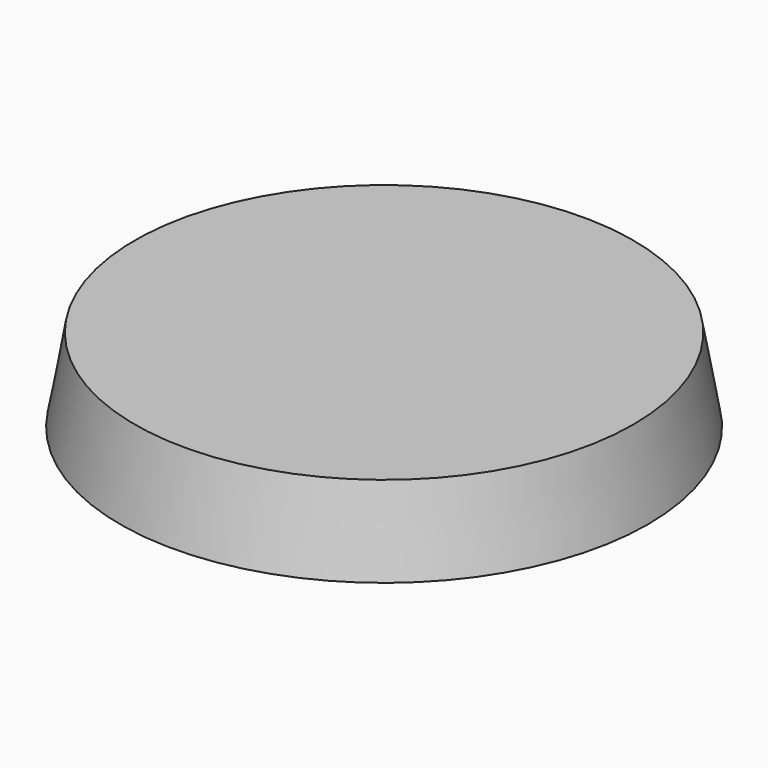
from build123d import *

# Parameters (mm, degrees)
F0_R           = 30
F1_DEPTH       = 10
F1_TAPER       = -10
F2_TEXT_SIZE   = 17.3544347483
F2_TEXT_SIZE_2 = 19.4131921465
F3_DEPTH       = 1


# Not quite as in the source:
# - Text() gives the source's letters only with a copy of the font that has no kerning and outlines rounded to 1/6400 em; it was checked with that copy


with BuildPart() as f1:
    # F0 (on Top) → F1 (new body)
    with BuildSketch(Plane.XY):
        Circle(F0_R)
    extrude(amount=-F1_DEPTH, taper=F1_TAPER)

    # F2 (on face) → F3 (cut)
    with BuildSketch(Plane(origin=(0, 0, -10), x_dir=(1, 0, 0), z_dir=(0, 0, -1))):
        with Locations((-27.5, 2.5048069812)):
            Text('Fredrik', F2_TEXT_SIZE, font='Open Sans', font_style=FontStyle.ITALIC, text_align=(TextAlign.LEFT, TextAlign.BOTTOM))
        with Locations((-27.5, -11.9774983455)):
            Text('Sanna', F2_TEXT_SIZE_2, font='Open Sans', font_style=FontStyle.ITALIC, text_align=(TextAlign.LEFT, TextAlign.BOTTOM))
    extrude(amount=-F3_DEPTH, mode=Mode.SUBTRACT)


solid = f1.part
